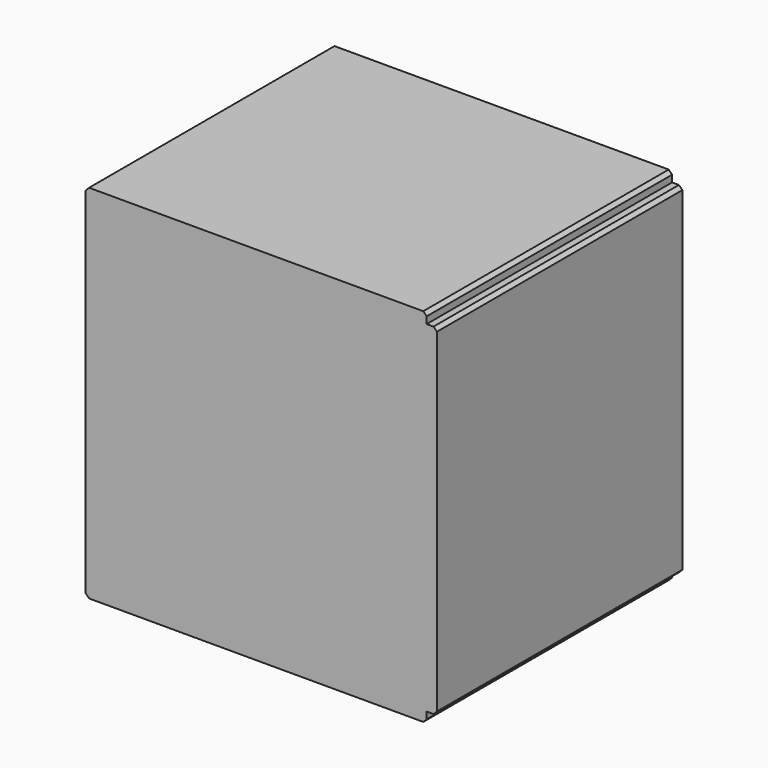
from build123d import *

# Parameters (mm, degrees)
F1_DEPTH = 26.98
F3_DEPTH = 26.98


# Not quite as in the source:
# - ends of sketch curves that miss each other by under 0.0002 mm in the source are joined


with BuildPart() as f1:
    # F0 (on Front) → F1 (new body)
    with BuildSketch(Plane.XZ):
        Polygon((0, 31.2), (0, 0), (29.991, 0), (29.991, 0.6005), (30.5914, 0.6005), (30.5914, 30.5996), (29.991, 30.5996), (29.991, 31.2), align=None)
    extrude(amount=F1_DEPTH)

    # F2 (on face) → F3 (join, through all)
    with BuildSketch(Plane.XZ.offset(26.98)):
        Polygon((0.3, 31.5), (0, 31.2), (29.991, 31.2), (29.691, 31.5), align=None)
        Polygon((30.8914, 30.2996), (30.5914, 30.5996), (30.5914, 0.6005), (30.8914480512, 0.9005009807), align=None)
        Polygon((29.991, 0), (0, 0), (0.3000519754, -0.2999990192), (29.6910519752, -0.2999029432), align=None)
    extrude(amount=-F3_DEPTH)


solid = f1.part
